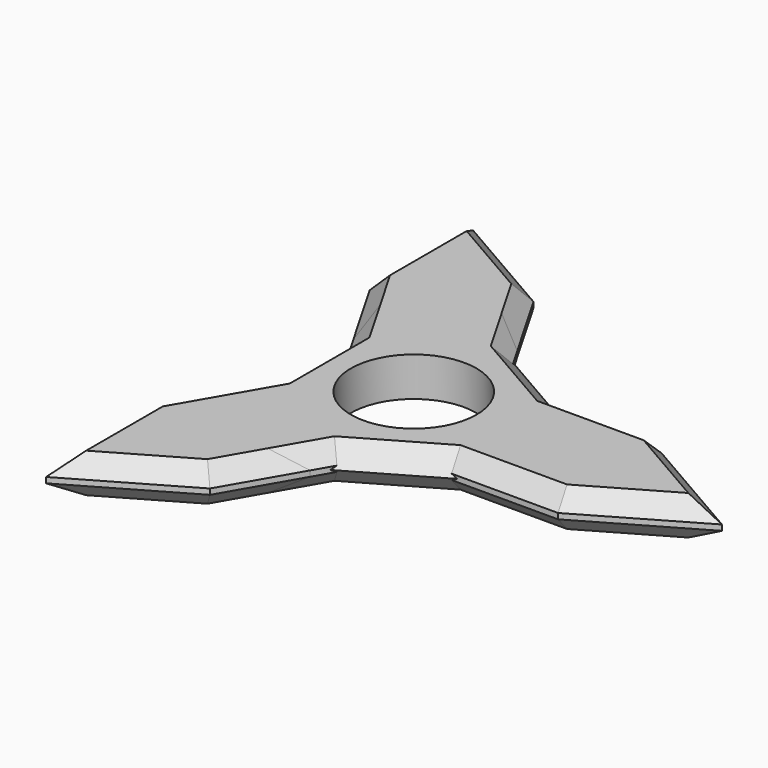
from build123d import *

# Parameters (mm, degrees)
F1_DEPTH      = 7
F2_SIZE       = 3
F3_T4_DEPTH   = 23.0940107676
F3_T10_DEPTH  = 23.0940107676
F3_T16_DEPTH  = 23.0940107676
F3_T22_DEPTH  = 23.0940107676
F3_T28_DEPTH  = 23.0940107676
F3_T34_DEPTH  = 23.0940107676
F3_T40_DEPTH  = 23.0940107676
F3_T46_DEPTH  = 23.0940107676
F3_T52_DEPTH  = 23.0940107676
F3_T58_DEPTH  = 23.0940107676
F3_T64_DEPTH  = 23.0940107676
F3_T70_DEPTH  = 23.0940107676
F3_T76_DEPTH  = 23.0940107676
F3_T82_DEPTH  = 23.0940107676
F3_T88_DEPTH  = 23.0940107676
F3_T94_DEPTH  = 23.0940107676
F3_T100_DEPTH = 23.0940107676
F3_T106_DEPTH = 23.0940107676
F3_T112_DEPTH = 23.0940107676
F3_T118_DEPTH = 23.0940107676
F3_T124_DEPTH = 23.0940107676
F3_T130_DEPTH = 23.0940107676
F3_T136_DEPTH = 23.0940107676
F3_T142_DEPTH = 23.0940107676
F3_T148_DEPTH = 18.8584149398
F3_T153_DEPTH = 18.8584149398
F3_T158_DEPTH = 18.8584149398
F3_T163_DEPTH = 18.8584149398
F3_T168_DEPTH = 18.8584149398
F3_T173_DEPTH = 18.8584149398
F3_T178_DEPTH = 18.8584149398
F3_T183_DEPTH = 18.8584149398
F3_T188_DEPTH = 18.8584149398
F3_T193_DEPTH = 18.8584149398
F3_T198_DEPTH = 18.8584149398
F3_T203_DEPTH = 18.8584149398
F3_T208_DEPTH = 18.8584149398
F3_T213_DEPTH = 18.8584149398
F3_T218_DEPTH = 18.8584149398
F3_T223_DEPTH = 18.8584149398
F3_T228_DEPTH = 18.8584149398
F3_T233_DEPTH = 18.8584149398
F3_T238_DEPTH = 18.8584149398
F3_T243_DEPTH = 18.8584149398
F3_T248_DEPTH = 18.8584149398
F3_T253_DEPTH = 18.8584149398
F3_T258_DEPTH = 18.8584149398
F3_T263_DEPTH = 18.8584149398


# Not quite as in the source:
# - a fillet or chamfer that OpenCascade refuses, or shapes differently, is made with other operations: its cross-section is extruded or revolved along the edge and cut away or added


with BuildPart() as f1:
    # F0 (on Top) → F1 (new body)
    with BuildSketch(Plane.XY):
        Polygon((-20, 11.5470053838), (-20, 0), (-20, -11.5470053838), (0, -23.0940107676), (20, -11.5470053838), (20, 11.5470053838), (0, 23.0940107676), align=None)
        with BuildLine():
            ThreePointArc((-11.2, 0), (0, 11.2), (11.2, 0))
            ThreePointArc((11.2, 0), (0, -11.2), (-11.2, 0))
        make_face(mode=Mode.SUBTRACT)
        Polygon((0, -23.0940107676), (-20, -11.5470053838), (-7.5, -36.0843918244), align=None)
        Polygon((-7.5, -36.0843918244), (-20, -11.5470053838), (-27.5, -24.5373864406), (-17.5, -30.3108891325), align=None)
        Polygon((-27.5, 24.5373864406), (-20, 11.5470053838), (0, 23.0940107676), align=None)
        Polygon((-27.5, -47.6313972081), (-7.5, -36.0843918244), (-17.5, -30.3108891325), align=None)
        Polygon((-17.5, -30.3108891325), (-27.5, -24.5373864406), (-27.5, -47.6313972081), align=None)
        Polygon((-27.5, 24.5373864406), (0, 23.0940107676), (-7.5, 36.0843918244), (-17.5, 30.3108891325), align=None)
        Polygon((-27.5, 47.6313972081), (-27.5, 24.5373864406), (-17.5, 30.3108891325), align=None)
        Polygon((20, 11.5470053838), (20, -11.5470053838), (35, 11.5470053838), align=None)
        Polygon((35, 11.5470053838), (20, -11.5470053838), (35, -11.5470053838), (35, 0), align=None)
        Polygon((-17.5, 30.3108891325), (-7.5, 36.0843918244), (-27.5, 47.6313972081), align=None)
        Polygon((55, 0), (35, 11.5470053838), (35, 0), align=None)
        Polygon((35, 0), (35, -11.5470053838), (55, 0), align=None)
    extrude(amount=F1_DEPTH)

    # F2
    f2_edges = [f1.edges().sort_by_distance(p)[0] for p in [
        (-27.5, 36.084392, 7),
        (-3.75, 29.589201, 7),
        (-23.75, 18.042196, 7),
        (-17.5, 41.857895, 7),
        (27.5, 11.547005, 7),
        (45, 5.773503, 7),
        (45, -5.773503, 7),
        (27.5, -11.547005, 7),
        (-3.75, -29.589201, 7),
        (-17.5, -41.857895, 7),
        (-27.5, -36.084392, 7),
        (-23.75, -18.042196, 7),
        (-17.5, 41.857895, 0),
        (-27.5, 36.084392, 0),
        (-3.75, 29.589201, 0),
        (-23.75, 18.042196, 0),
        (-23.75, -18.042196, 0),
        (-27.5, -36.084392, 0),
        (-17.5, -41.857895, 0),
        (-3.75, -29.589201, 0),
        (27.5, -11.547005, 0),
        (45, -5.773503, 0),
        (45, 5.773503, 0),
        (27.5, 11.547005, 0),
    ]]
    chamfer(f2_edges, length=F2_SIZE)

    # F3: chamfer of 5 on 6 edges, made by hand


with BuildPart() as f3_tool2:
    # F3_s3 → F3_t4 (new body)
    with BuildSketch(Plane(origin=(10, -5.7735026919, 0), x_dir=(0, 0, 1), z_dir=(-0.8660254038, 0.5, 0))):
        Polygon((0, 15), (5, 20), (0, 20), align=None)
    extrude(amount=F3_T4_DEPTH)

    split(bisect_by=Plane(origin=(0, 7.7735026919, 7.7735026919), x_dir=(1, 0, 0), z_dir=(0, 0.7071067812, 0.7071067812)), keep=Keep.TOP)

    split(bisect_by=Plane(origin=(10, 5.7735026919, 0), x_dir=(0, 0, 1), z_dir=(0.8660254038, 0.5, 0)), keep=Keep.TOP)


with BuildPart() as f1_1:
    add(f1.part)

    # F3_t1: cut F3_tool2
    add(f3_tool2.part, mode=Mode.SUBTRACT)


with BuildPart() as f3_tool8:
    # F3_s9 → F3_t10 (new body)
    with BuildSketch(Plane(origin=(10, -5.7735026919, 0), x_dir=(0, 0, 1), z_dir=(-0.8660254038, 0.5, 0))):
        Polygon((0, 15), (5, 20), (0, 20), align=None)
    extrude(amount=F3_T10_DEPTH)

    split(bisect_by=Plane(origin=(3.7009618943, 2.1367513459, -4.2735026919), x_dir=(-0.5, 0.8660254038, 0), z_dir=(0.6123724357, 0.3535533906, -0.7071067812)), keep=Keep.TOP)

    split(bisect_by=Plane.XZ.offset(-11.5470053838), keep=Keep.BOTTOM)


with BuildPart() as f1_2:
    add(f1_1.part)

    # F3_t7: cut F3_tool8
    add(f3_tool8.part, mode=Mode.SUBTRACT)


with BuildPart() as f3_tool14:
    # F3_s15 → F3_t16 (new body)
    with BuildSketch(Plane(origin=(10, -5.7735026919, 0), x_dir=(0, 0, 1), z_dir=(-0.8660254038, 0.5, 0))):
        Polygon((0, 15), (5, 20), (0, 20), align=None)
    extrude(amount=F3_T16_DEPTH)

    split(bisect_by=Plane(origin=(0, 4.2735026919, -4.2735026919), x_dir=(1, 0, 0), z_dir=(0, 0.7071067812, -0.7071067812)), keep=Keep.TOP)

    split(bisect_by=Plane(origin=(10, 5.7735026919, 0), x_dir=(0, 0, 1), z_dir=(0.8660254038, 0.5, 0)), keep=Keep.TOP)


with BuildPart() as f1_3:
    add(f1_2.part)

    # F3_t13: cut F3_tool14
    add(f3_tool14.part, mode=Mode.SUBTRACT)


with BuildPart() as f3_tool20:
    # F3_s21 → F3_t22 (new body)
    with BuildSketch(Plane(origin=(10, -5.7735026919, 0), x_dir=(0, 0, 1), z_dir=(-0.8660254038, 0.5, 0))):
        Polygon((0, 15), (5, 20), (0, 20), align=None)
    extrude(amount=F3_T22_DEPTH)

    split(bisect_by=Plane(origin=(6.7320508076, 3.8867513459, 7.7735026919), x_dir=(-0.5, 0.8660254038, 0), z_dir=(0.6123724357, 0.3535533906, 0.7071067812)), keep=Keep.TOP)

    split(bisect_by=Plane(origin=(10, 5.7735026919, 0), x_dir=(0, 0, 1), z_dir=(-0.8660254038, -0.5, 0)), keep=Keep.TOP)


with BuildPart() as f1_4:
    add(f1_3.part)

    # F3_t19: cut F3_tool20
    add(f3_tool20.part, mode=Mode.SUBTRACT)


with BuildPart() as f3_tool26:
    # F3_s27 → F3_t28 (new body)
    with BuildSketch(Plane.XZ.offset(-11.5470053838)):
        Polygon((-20, 5), (-15, 0), (-20, 0), align=None)
    extrude(amount=F3_T28_DEPTH)

    split(bisect_by=Plane(origin=(-10, -5.7735026919, 0), x_dir=(0, 0, 1), z_dir=(-0.8660254038, -0.5, 0)), keep=Keep.TOP)

    split(bisect_by=Plane(origin=(-10, 5.7735026919, 0), x_dir=(0, 0, 1), z_dir=(-0.8660254038, 0.5, 0)), keep=Keep.TOP)


with BuildPart() as f1_5:
    add(f1_4.part)

    # F3_t25: cut F3_tool26
    add(f3_tool26.part, mode=Mode.SUBTRACT)


with BuildPart() as f3_tool32:
    # F3_s33 → F3_t34 (new body)
    with BuildSketch(Plane.XZ.offset(-11.5470053838)):
        Polygon((-20, 5), (-15, 0), (-20, 0), align=None)
    extrude(amount=F3_T34_DEPTH)

    split(bisect_by=Plane(origin=(-6.7320508076, -3.8867513459, 7.7735026919), x_dir=(0.5, -0.8660254038, 0), z_dir=(-0.6123724357, -0.3535533906, 0.7071067812)), keep=Keep.TOP)

    split(bisect_by=Plane(origin=(-3.7009618943, 2.1367513459, -4.2735026919), x_dir=(-0.5, -0.8660254038, 0), z_dir=(-0.6123724357, 0.3535533906, -0.7071067812)), keep=Keep.TOP)


with BuildPart() as f1_6:
    add(f1_5.part)

    # F3_t31: cut F3_tool32
    add(f3_tool32.part, mode=Mode.SUBTRACT)


with BuildPart() as f3_tool38:
    # F3_s39 → F3_t40 (new body)
    with BuildSketch(Plane.XZ.offset(-11.5470053838)):
        Polygon((-20, 5), (-15, 0), (-20, 0), align=None)
    extrude(amount=F3_T40_DEPTH)

    split(bisect_by=Plane(origin=(-3.7009618943, -2.1367513459, -4.2735026919), x_dir=(0.5, -0.8660254038, 0), z_dir=(-0.6123724357, -0.3535533906, -0.7071067812)), keep=Keep.TOP)

    split(bisect_by=Plane(origin=(-3.7009618943, 2.1367513459, -4.2735026919), x_dir=(-0.5, -0.8660254038, 0), z_dir=(-0.6123724357, 0.3535533906, -0.7071067812)), keep=Keep.TOP)


with BuildPart() as f1_7:
    add(f1_6.part)

    # F3_t37: cut F3_tool38
    add(f3_tool38.part, mode=Mode.SUBTRACT)


with BuildPart() as f3_tool44:
    # F3_s45 → F3_t46 (new body)
    with BuildSketch(Plane.XZ.offset(-11.5470053838)):
        Polygon((-20, 5), (-15, 0), (-20, 0), align=None)
    extrude(amount=F3_T46_DEPTH)

    split(bisect_by=Plane(origin=(-6.7320508076, 3.8867513459, 7.7735026919), x_dir=(-0.5, -0.8660254038, 0), z_dir=(-0.6123724357, 0.3535533906, 0.7071067812)), keep=Keep.TOP)

    split(bisect_by=Plane(origin=(-10, 5.7735026919, 0), x_dir=(0, 0, 1), z_dir=(0.8660254038, -0.5, 0)), keep=Keep.TOP)


with BuildPart() as f1_8:
    add(f1_7.part)

    # F3_t43: cut F3_tool44
    add(f3_tool44.part, mode=Mode.SUBTRACT)


with BuildPart() as f3_tool50:
    # F3_s51 → F3_t52 (new body)
    with BuildSketch(Plane(origin=(-10, -5.7735026919, 0), x_dir=(0, 0, 1), z_dir=(0.8660254038, 0.5, 0))):
        Polygon((0, 15), (5, 20), (0, 20), align=None)
    extrude(amount=F3_T52_DEPTH)

    split(bisect_by=Plane(origin=(6.7320508076, -3.8867513459, 7.7735026919), x_dir=(0.5, 0.8660254038, 0), z_dir=(0.6123724357, -0.3535533906, 0.7071067812)), keep=Keep.TOP)

    split(bisect_by=Plane.XZ.offset(11.5470053838), keep=Keep.TOP)


with BuildPart() as f1_9:
    add(f1_8.part)

    # F3_t49: cut F3_tool50
    add(f3_tool50.part, mode=Mode.SUBTRACT)


with BuildPart() as f3_tool56:
    # F3_s57 → F3_t58 (new body)
    with BuildSketch(Plane(origin=(-10, -5.7735026919, 0), x_dir=(0, 0, 1), z_dir=(0.8660254038, 0.5, 0))):
        Polygon((0, 15), (5, 20), (0, 20), align=None)
    extrude(amount=F3_T58_DEPTH)

    split(bisect_by=Plane(origin=(0, -4.2735026919, -4.2735026919), x_dir=(1, 0, 0), z_dir=(0, -0.7071067812, -0.7071067812)), keep=Keep.TOP)

    split(bisect_by=Plane(origin=(10, -5.7735026919, 0), x_dir=(0, 0, 1), z_dir=(0.8660254038, -0.5, 0)), keep=Keep.TOP)


with BuildPart() as f1_10:
    add(f1_9.part)

    # F3_t55: cut F3_tool56
    add(f3_tool56.part, mode=Mode.SUBTRACT)


with BuildPart() as f3_tool62:
    # F3_s63 → F3_t64 (new body)
    with BuildSketch(Plane(origin=(-10, -5.7735026919, 0), x_dir=(0, 0, 1), z_dir=(0.8660254038, 0.5, 0))):
        Polygon((0, 15), (5, 20), (0, 20), align=None)
    extrude(amount=F3_T64_DEPTH)

    split(bisect_by=Plane(origin=(3.7009618943, -2.1367513459, -4.2735026919), x_dir=(0.5, 0.8660254038, 0), z_dir=(0.6123724357, -0.3535533906, -0.7071067812)), keep=Keep.TOP)

    split(bisect_by=Plane(origin=(10, -5.7735026919, 0), x_dir=(0, 0, 1), z_dir=(-0.8660254038, 0.5, 0)), keep=Keep.TOP)


with BuildPart() as f1_11:
    add(f1_10.part)

    # F3_t61: cut F3_tool62
    add(f3_tool62.part, mode=Mode.SUBTRACT)


with BuildPart() as f3_tool68:
    # F3_s69 → F3_t70 (new body)
    with BuildSketch(Plane(origin=(-10, -5.7735026919, 0), x_dir=(0, 0, 1), z_dir=(0.8660254038, 0.5, 0))):
        Polygon((0, 15), (5, 20), (0, 20), align=None)
    extrude(amount=F3_T70_DEPTH)

    split(bisect_by=Plane(origin=(0, -7.7735026919, 7.7735026919), x_dir=(1, 0, 0), z_dir=(0, -0.7071067812, 0.7071067812)), keep=Keep.TOP)

    split(bisect_by=Plane(origin=(10, -5.7735026919, 0), x_dir=(0, 0, 1), z_dir=(0.8660254038, -0.5, 0)), keep=Keep.TOP)


with BuildPart() as f1_12:
    add(f1_11.part)

    # F3_t67: cut F3_tool68
    add(f3_tool68.part, mode=Mode.SUBTRACT)


with BuildPart() as f3_tool74:
    # F3_s75 → F3_t76 (new body)
    with BuildSketch(Plane.XZ.offset(-11.5470053838)):
        Polygon((-20, 2), (-15, 7), (-20, 7), align=None)
    extrude(amount=F3_T76_DEPTH)

    split(bisect_by=Plane(origin=(-10, -5.7735026919, 0), x_dir=(0, 0, 1), z_dir=(-0.8660254038, -0.5, 0)), keep=Keep.TOP)

    split(bisect_by=Plane(origin=(-10, 5.7735026919, 0), x_dir=(0, 0, 1), z_dir=(-0.8660254038, 0.5, 0)), keep=Keep.TOP)


with BuildPart() as f1_13:
    add(f1_12.part)

    # F3_t73: cut F3_tool74
    add(f3_tool74.part, mode=Mode.SUBTRACT)


with BuildPart() as f3_tool80:
    # F3_s81 → F3_t82 (new body)
    with BuildSketch(Plane.XZ.offset(-11.5470053838)):
        Polygon((-20, 2), (-15, 7), (-20, 7), align=None)
    extrude(amount=F3_T82_DEPTH)

    split(bisect_by=Plane(origin=(-3.7009618943, -2.1367513459, -4.2735026919), x_dir=(0.5, -0.8660254038, 0), z_dir=(-0.6123724357, -0.3535533906, -0.7071067812)), keep=Keep.TOP)

    split(bisect_by=Plane(origin=(-6.7320508076, 3.8867513459, 7.7735026919), x_dir=(-0.5, -0.8660254038, 0), z_dir=(-0.6123724357, 0.3535533906, 0.7071067812)), keep=Keep.TOP)


with BuildPart() as f1_14:
    add(f1_13.part)

    # F3_t79: cut F3_tool80
    add(f3_tool80.part, mode=Mode.SUBTRACT)


with BuildPart() as f3_tool86:
    # F3_s87 → F3_t88 (new body)
    with BuildSketch(Plane.XZ.offset(-11.5470053838)):
        Polygon((-20, 2), (-15, 7), (-20, 7), align=None)
    extrude(amount=F3_T88_DEPTH)

    split(bisect_by=Plane(origin=(-6.7320508076, -3.8867513459, 7.7735026919), x_dir=(0.5, -0.8660254038, 0), z_dir=(-0.6123724357, -0.3535533906, 0.7071067812)), keep=Keep.TOP)

    split(bisect_by=Plane(origin=(-6.7320508076, 3.8867513459, 7.7735026919), x_dir=(-0.5, -0.8660254038, 0), z_dir=(-0.6123724357, 0.3535533906, 0.7071067812)), keep=Keep.TOP)


with BuildPart() as f1_15:
    add(f1_14.part)

    # F3_t85: cut F3_tool86
    add(f3_tool86.part, mode=Mode.SUBTRACT)


with BuildPart() as f3_tool92:
    # F3_s93 → F3_t94 (new body)
    with BuildSketch(Plane.XZ.offset(-11.5470053838)):
        Polygon((-20, 2), (-15, 7), (-20, 7), align=None)
    extrude(amount=F3_T94_DEPTH)

    split(bisect_by=Plane(origin=(-3.7009618943, 2.1367513459, -4.2735026919), x_dir=(-0.5, -0.8660254038, 0), z_dir=(-0.6123724357, 0.3535533906, -0.7071067812)), keep=Keep.TOP)

    split(bisect_by=Plane(origin=(-10, 5.7735026919, 0), x_dir=(0, 0, 1), z_dir=(0.8660254038, -0.5, 0)), keep=Keep.TOP)


with BuildPart() as f1_16:
    add(f1_15.part)

    # F3_t91: cut F3_tool92
    add(f3_tool92.part, mode=Mode.SUBTRACT)


with BuildPart() as f3_tool98:
    # F3_s99 → F3_t100 (new body)
    with BuildSketch(Plane(origin=(10, -5.7735026919, 0), x_dir=(0, 0, 1), z_dir=(-0.8660254038, 0.5, 0))):
        Polygon((7, 15), (2, 20), (7, 20), align=None)
    extrude(amount=F3_T100_DEPTH)

    split(bisect_by=Plane(origin=(0, 4.2735026919, -4.2735026919), x_dir=(1, 0, 0), z_dir=(0, 0.7071067812, -0.7071067812)), keep=Keep.TOP)

    split(bisect_by=Plane(origin=(10, 5.7735026919, 0), x_dir=(0, 0, 1), z_dir=(0.8660254038, 0.5, 0)), keep=Keep.TOP)


with BuildPart() as f1_17:
    add(f1_16.part)

    # F3_t97: cut F3_tool98
    add(f3_tool98.part, mode=Mode.SUBTRACT)


with BuildPart() as f3_tool104:
    # F3_s105 → F3_t106 (new body)
    with BuildSketch(Plane(origin=(10, -5.7735026919, 0), x_dir=(0, 0, 1), z_dir=(-0.8660254038, 0.5, 0))):
        Polygon((7, 15), (2, 20), (7, 20), align=None)
    extrude(amount=F3_T106_DEPTH)

    split(bisect_by=Plane(origin=(6.7320508076, 3.8867513459, 7.7735026919), x_dir=(-0.5, 0.8660254038, 0), z_dir=(0.6123724357, 0.3535533906, 0.7071067812)), keep=Keep.TOP)

    split(bisect_by=Plane.XZ.offset(-11.5470053838), keep=Keep.BOTTOM)


with BuildPart() as f1_18:
    add(f1_17.part)

    # F3_t103: cut F3_tool104
    add(f3_tool104.part, mode=Mode.SUBTRACT)


with BuildPart() as f3_tool110:
    # F3_s111 → F3_t112 (new body)
    with BuildSketch(Plane(origin=(10, -5.7735026919, 0), x_dir=(0, 0, 1), z_dir=(-0.8660254038, 0.5, 0))):
        Polygon((7, 15), (2, 20), (7, 20), align=None)
    extrude(amount=F3_T112_DEPTH)

    split(bisect_by=Plane(origin=(0, 7.7735026919, 7.7735026919), x_dir=(1, 0, 0), z_dir=(0, 0.7071067812, 0.7071067812)), keep=Keep.TOP)

    split(bisect_by=Plane(origin=(10, 5.7735026919, 0), x_dir=(0, 0, 1), z_dir=(0.8660254038, 0.5, 0)), keep=Keep.TOP)


with BuildPart() as f1_19:
    add(f1_18.part)

    # F3_t109: cut F3_tool110
    add(f3_tool110.part, mode=Mode.SUBTRACT)


with BuildPart() as f3_tool116:
    # F3_s117 → F3_t118 (new body)
    with BuildSketch(Plane(origin=(10, -5.7735026919, 0), x_dir=(0, 0, 1), z_dir=(-0.8660254038, 0.5, 0))):
        Polygon((7, 15), (2, 20), (7, 20), align=None)
    extrude(amount=F3_T118_DEPTH)

    split(bisect_by=Plane(origin=(3.7009618943, 2.1367513459, -4.2735026919), x_dir=(-0.5, 0.8660254038, 0), z_dir=(0.6123724357, 0.3535533906, -0.7071067812)), keep=Keep.TOP)

    split(bisect_by=Plane(origin=(10, 5.7735026919, 0), x_dir=(0, 0, 1), z_dir=(-0.8660254038, -0.5, 0)), keep=Keep.TOP)


with BuildPart() as f1_20:
    add(f1_19.part)

    # F3_t115: cut F3_tool116
    add(f3_tool116.part, mode=Mode.SUBTRACT)


with BuildPart() as f3_tool122:
    # F3_s123 → F3_t124 (new body)
    with BuildSketch(Plane(origin=(-10, -5.7735026919, 0), x_dir=(0, 0, 1), z_dir=(0.8660254038, 0.5, 0))):
        Polygon((7, 15), (2, 20), (7, 20), align=None)
    extrude(amount=F3_T124_DEPTH)

    split(bisect_by=Plane(origin=(3.7009618943, -2.1367513459, -4.2735026919), x_dir=(0.5, 0.8660254038, 0), z_dir=(0.6123724357, -0.3535533906, -0.7071067812)), keep=Keep.TOP)

    split(bisect_by=Plane.XZ.offset(11.5470053838), keep=Keep.TOP)


with BuildPart() as f1_21:
    add(f1_20.part)

    # F3_t121: cut F3_tool122
    add(f3_tool122.part, mode=Mode.SUBTRACT)


with BuildPart() as f3_tool128:
    # F3_s129 → F3_t130 (new body)
    with BuildSketch(Plane(origin=(-10, -5.7735026919, 0), x_dir=(0, 0, 1), z_dir=(0.8660254038, 0.5, 0))):
        Polygon((7, 15), (2, 20), (7, 20), align=None)
    extrude(amount=F3_T130_DEPTH)

    split(bisect_by=Plane(origin=(0, -7.7735026919, 7.7735026919), x_dir=(1, 0, 0), z_dir=(0, -0.7071067812, 0.7071067812)), keep=Keep.TOP)

    split(bisect_by=Plane(origin=(10, -5.7735026919, 0), x_dir=(0, 0, 1), z_dir=(0.8660254038, -0.5, 0)), keep=Keep.TOP)


with BuildPart() as f1_22:
    add(f1_21.part)

    # F3_t127: cut F3_tool128
    add(f3_tool128.part, mode=Mode.SUBTRACT)


with BuildPart() as f3_tool134:
    # F3_s135 → F3_t136 (new body)
    with BuildSketch(Plane(origin=(-10, -5.7735026919, 0), x_dir=(0, 0, 1), z_dir=(0.8660254038, 0.5, 0))):
        Polygon((7, 15), (2, 20), (7, 20), align=None)
    extrude(amount=F3_T136_DEPTH)

    split(bisect_by=Plane(origin=(6.7320508076, -3.8867513459, 7.7735026919), x_dir=(0.5, 0.8660254038, 0), z_dir=(0.6123724357, -0.3535533906, 0.7071067812)), keep=Keep.TOP)

    split(bisect_by=Plane(origin=(10, -5.7735026919, 0), x_dir=(0, 0, 1), z_dir=(-0.8660254038, 0.5, 0)), keep=Keep.TOP)


with BuildPart() as f1_23:
    add(f1_22.part)

    # F3_t133: cut F3_tool134
    add(f3_tool134.part, mode=Mode.SUBTRACT)


with BuildPart() as f3_tool140:
    # F3_s141 → F3_t142 (new body)
    with BuildSketch(Plane(origin=(-10, -5.7735026919, 0), x_dir=(0, 0, 1), z_dir=(0.8660254038, 0.5, 0))):
        Polygon((7, 15), (2, 20), (7, 20), align=None)
    extrude(amount=F3_T142_DEPTH)

    split(bisect_by=Plane(origin=(0, -4.2735026919, -4.2735026919), x_dir=(1, 0, 0), z_dir=(0, -0.7071067812, -0.7071067812)), keep=Keep.TOP)

    split(bisect_by=Plane(origin=(10, -5.7735026919, 0), x_dir=(0, 0, 1), z_dir=(0.8660254038, -0.5, 0)), keep=Keep.TOP)


with BuildPart() as f1_24:
    add(f1_23.part)

    # F3_t139: cut F3_tool140
    add(f3_tool140.part, mode=Mode.SUBTRACT)


with BuildPart() as f3_tool146:
    # F3_s147 → F3_t148 (new body)
    with BuildSketch(Plane(origin=(-10, -5.7735026919, 0), x_dir=(0, 0, 1), z_dir=(-0.8660254038, -0.5, 0))):
        Polygon((7, -15), (2, -20), (7, -20), align=None)
    extrude(amount=F3_T148_DEPTH)

    split(bisect_by=Plane(origin=(3.7009618943, -2.1367513459, -4.2735026919), x_dir=(0.5, 0.8660254038, 0), z_dir=(0.6123724357, -0.3535533906, -0.7071067812)), keep=Keep.TOP)


with BuildPart() as f1_25:
    add(f1_24.part)

    # F3_t145: cut F3_tool146
    add(f3_tool146.part, mode=Mode.SUBTRACT)


with BuildPart() as f3_tool151:
    # F3_s152 → F3_t153 (new body)
    with BuildSketch(Plane(origin=(-10, -5.7735026919, 0), x_dir=(0, 0, 1), z_dir=(-0.8660254038, -0.5, 0))):
        Polygon((7, -15), (2, -20), (7, -20), align=None)
    extrude(amount=F3_T153_DEPTH)

    split(bisect_by=Plane(origin=(6.7320508076, -3.8867513459, 7.7735026919), x_dir=(0.5, 0.8660254038, 0), z_dir=(0.6123724357, -0.3535533906, 0.7071067812)), keep=Keep.TOP)


with BuildPart() as f1_26:
    add(f1_25.part)

    # F3_t150: cut F3_tool151
    add(f3_tool151.part, mode=Mode.SUBTRACT)


with BuildPart() as f3_tool156:
    # F3_s157 → F3_t158 (new body)
    with BuildSketch(Plane(origin=(10, 5.7735026919, 0), x_dir=(0, 0, 1), z_dir=(0.8660254038, 0.5, 0))):
        Polygon((7, 15), (2, 20), (7, 20), align=None)
    extrude(amount=F3_T158_DEPTH)

    split(bisect_by=Plane(origin=(0, -4.2735026919, -4.2735026919), x_dir=(1, 0, 0), z_dir=(0, -0.7071067812, -0.7071067812)), keep=Keep.TOP)


with BuildPart() as f1_27:
    add(f1_26.part)

    # F3_t155: cut F3_tool156
    add(f3_tool156.part, mode=Mode.SUBTRACT)


with BuildPart() as f3_tool161:
    # F3_s162 → F3_t163 (new body)
    with BuildSketch(Plane(origin=(10, 5.7735026919, 0), x_dir=(0, 0, 1), z_dir=(0.8660254038, 0.5, 0))):
        Polygon((7, 15), (2, 20), (7, 20), align=None)
    extrude(amount=F3_T163_DEPTH)

    split(bisect_by=Plane(origin=(0, -7.7735026919, 7.7735026919), x_dir=(1, 0, 0), z_dir=(0, -0.7071067812, 0.7071067812)), keep=Keep.TOP)


with BuildPart() as f1_28:
    add(f1_27.part)

    # F3_t160: cut F3_tool161
    add(f3_tool161.part, mode=Mode.SUBTRACT)


with BuildPart() as f3_tool166:
    # F3_s167 → F3_t168 (new body)
    with BuildSketch(Plane(origin=(10, -5.7735026919, 0), x_dir=(0, 0, 1), z_dir=(0.8660254038, -0.5, 0))):
        Polygon((7, -15), (2, -20), (7, -20), align=None)
    extrude(amount=F3_T168_DEPTH)

    split(bisect_by=Plane(origin=(0, 4.2735026919, -4.2735026919), x_dir=(1, 0, 0), z_dir=(0, 0.7071067812, -0.7071067812)), keep=Keep.TOP)


with BuildPart() as f1_29:
    add(f1_28.part)

    # F3_t165: cut F3_tool166
    add(f3_tool166.part, mode=Mode.SUBTRACT)


with BuildPart() as f3_tool171:
    # F3_s172 → F3_t173 (new body)
    with BuildSketch(Plane(origin=(10, -5.7735026919, 0), x_dir=(0, 0, 1), z_dir=(0.8660254038, -0.5, 0))):
        Polygon((7, -15), (2, -20), (7, -20), align=None)
    extrude(amount=F3_T173_DEPTH)

    split(bisect_by=Plane(origin=(0, 7.7735026919, 7.7735026919), x_dir=(1, 0, 0), z_dir=(0, 0.7071067812, 0.7071067812)), keep=Keep.TOP)


with BuildPart() as f1_30:
    add(f1_29.part)

    # F3_t170: cut F3_tool171
    add(f3_tool171.part, mode=Mode.SUBTRACT)


with BuildPart() as f3_tool176:
    # F3_s177 → F3_t178 (new body)
    with BuildSketch(Plane(origin=(-10, 5.7735026919, 0), x_dir=(0, 0, 1), z_dir=(-0.8660254038, 0.5, 0))):
        Polygon((7, 15), (2, 20), (7, 20), align=None)
    extrude(amount=F3_T178_DEPTH)

    split(bisect_by=Plane(origin=(3.7009618943, 2.1367513459, -4.2735026919), x_dir=(-0.5, 0.8660254038, 0), z_dir=(0.6123724357, 0.3535533906, -0.7071067812)), keep=Keep.TOP)


with BuildPart() as f1_31:
    add(f1_30.part)

    # F3_t175: cut F3_tool176
    add(f3_tool176.part, mode=Mode.SUBTRACT)


with BuildPart() as f3_tool181:
    # F3_s182 → F3_t183 (new body)
    with BuildSketch(Plane(origin=(-10, 5.7735026919, 0), x_dir=(0, 0, 1), z_dir=(-0.8660254038, 0.5, 0))):
        Polygon((7, 15), (2, 20), (7, 20), align=None)
    extrude(amount=F3_T183_DEPTH)

    split(bisect_by=Plane(origin=(6.7320508076, 3.8867513459, 7.7735026919), x_dir=(-0.5, 0.8660254038, 0), z_dir=(0.6123724357, 0.3535533906, 0.7071067812)), keep=Keep.TOP)


with BuildPart() as f1_32:
    add(f1_31.part)

    # F3_t180: cut F3_tool181
    add(f3_tool181.part, mode=Mode.SUBTRACT)


with BuildPart() as f3_tool186:
    # F3_s187 → F3_t188 (new body)
    with BuildSketch(Plane.XZ.offset(-11.5470053838)):
        Polygon((-20, 2), (-15, 7), (-20, 7), align=None)
    extrude(amount=-F3_T188_DEPTH)

    split(bisect_by=Plane(origin=(-3.7009618943, -2.1367513459, -4.2735026919), x_dir=(0.5, -0.8660254038, 0), z_dir=(-0.6123724357, -0.3535533906, -0.7071067812)), keep=Keep.TOP)


with BuildPart() as f1_33:
    add(f1_32.part)

    # F3_t185: cut F3_tool186
    add(f3_tool186.part, mode=Mode.SUBTRACT)


with BuildPart() as f3_tool191:
    # F3_s192 → F3_t193 (new body)
    with BuildSketch(Plane.XZ.offset(-11.5470053838)):
        Polygon((-20, 2), (-15, 7), (-20, 7), align=None)
    extrude(amount=-F3_T193_DEPTH)

    split(bisect_by=Plane(origin=(-6.7320508076, -3.8867513459, 7.7735026919), x_dir=(0.5, -0.8660254038, 0), z_dir=(-0.6123724357, -0.3535533906, 0.7071067812)), keep=Keep.TOP)


with BuildPart() as f1_34:
    add(f1_33.part)

    # F3_t190: cut F3_tool191
    add(f3_tool191.part, mode=Mode.SUBTRACT)


with BuildPart() as f3_tool196:
    # F3_s197 → F3_t198 (new body)
    with BuildSketch(Plane.XZ.offset(11.5470053838)):
        Polygon((-20, 2), (-15, 7), (-20, 7), align=None)
    extrude(amount=F3_T198_DEPTH)

    split(bisect_by=Plane(origin=(-3.7009618943, 2.1367513459, -4.2735026919), x_dir=(-0.5, -0.8660254038, 0), z_dir=(-0.6123724357, 0.3535533906, -0.7071067812)), keep=Keep.TOP)


with BuildPart() as f1_35:
    add(f1_34.part)

    # F3_t195: cut F3_tool196
    add(f3_tool196.part, mode=Mode.SUBTRACT)


with BuildPart() as f3_tool201:
    # F3_s202 → F3_t203 (new body)
    with BuildSketch(Plane.XZ.offset(11.5470053838)):
        Polygon((-20, 2), (-15, 7), (-20, 7), align=None)
    extrude(amount=F3_T203_DEPTH)

    split(bisect_by=Plane(origin=(-6.7320508076, 3.8867513459, 7.7735026919), x_dir=(-0.5, -0.8660254038, 0), z_dir=(-0.6123724357, 0.3535533906, 0.7071067812)), keep=Keep.TOP)


with BuildPart() as f1_36:
    add(f1_35.part)

    # F3_t200: cut F3_tool201
    add(f3_tool201.part, mode=Mode.SUBTRACT)


with BuildPart() as f3_tool206:
    # F3_s207 → F3_t208 (new body)
    with BuildSketch(Plane(origin=(-10, -5.7735026919, 0), x_dir=(0, 0, 1), z_dir=(-0.8660254038, -0.5, 0))):
        Polygon((0, -15), (5, -20), (0, -20), align=None)
    extrude(amount=F3_T208_DEPTH)

    split(bisect_by=Plane(origin=(6.7320508076, -3.8867513459, 7.7735026919), x_dir=(0.5, 0.8660254038, 0), z_dir=(0.6123724357, -0.3535533906, 0.7071067812)), keep=Keep.TOP)


with BuildPart() as f1_37:
    add(f1_36.part)

    # F3_t205: cut F3_tool206
    add(f3_tool206.part, mode=Mode.SUBTRACT)


with BuildPart() as f3_tool211:
    # F3_s212 → F3_t213 (new body)
    with BuildSketch(Plane(origin=(-10, -5.7735026919, 0), x_dir=(0, 0, 1), z_dir=(-0.8660254038, -0.5, 0))):
        Polygon((0, -15), (5, -20), (0, -20), align=None)
    extrude(amount=F3_T213_DEPTH)

    split(bisect_by=Plane(origin=(3.7009618943, -2.1367513459, -4.2735026919), x_dir=(0.5, 0.8660254038, 0), z_dir=(0.6123724357, -0.3535533906, -0.7071067812)), keep=Keep.TOP)


with BuildPart() as f1_38:
    add(f1_37.part)

    # F3_t210: cut F3_tool211
    add(f3_tool211.part, mode=Mode.SUBTRACT)


with BuildPart() as f3_tool216:
    # F3_s217 → F3_t218 (new body)
    with BuildSketch(Plane(origin=(10, 5.7735026919, 0), x_dir=(0, 0, 1), z_dir=(0.8660254038, 0.5, 0))):
        Polygon((0, 15), (5, 20), (0, 20), align=None)
    extrude(amount=F3_T218_DEPTH)

    split(bisect_by=Plane(origin=(0, -7.7735026919, 7.7735026919), x_dir=(1, 0, 0), z_dir=(0, -0.7071067812, 0.7071067812)), keep=Keep.TOP)


with BuildPart() as f1_39:
    add(f1_38.part)

    # F3_t215: cut F3_tool216
    add(f3_tool216.part, mode=Mode.SUBTRACT)


with BuildPart() as f3_tool221:
    # F3_s222 → F3_t223 (new body)
    with BuildSketch(Plane(origin=(10, 5.7735026919, 0), x_dir=(0, 0, 1), z_dir=(0.8660254038, 0.5, 0))):
        Polygon((0, 15), (5, 20), (0, 20), align=None)
    extrude(amount=F3_T223_DEPTH)

    split(bisect_by=Plane(origin=(0, -4.2735026919, -4.2735026919), x_dir=(1, 0, 0), z_dir=(0, -0.7071067812, -0.7071067812)), keep=Keep.TOP)


with BuildPart() as f1_40:
    add(f1_39.part)

    # F3_t220: cut F3_tool221
    add(f3_tool221.part, mode=Mode.SUBTRACT)


with BuildPart() as f3_tool226:
    # F3_s227 → F3_t228 (new body)
    with BuildSketch(Plane.XZ.offset(-11.5470053838)):
        Polygon((-20, 5), (-15, 0), (-20, 0), align=None)
    extrude(amount=-F3_T228_DEPTH)

    split(bisect_by=Plane(origin=(-6.7320508076, -3.8867513459, 7.7735026919), x_dir=(0.5, -0.8660254038, 0), z_dir=(-0.6123724357, -0.3535533906, 0.7071067812)), keep=Keep.TOP)


with BuildPart() as f1_41:
    add(f1_40.part)

    # F3_t225: cut F3_tool226
    add(f3_tool226.part, mode=Mode.SUBTRACT)


with BuildPart() as f3_tool231:
    # F3_s232 → F3_t233 (new body)
    with BuildSketch(Plane.XZ.offset(-11.5470053838)):
        Polygon((-20, 5), (-15, 0), (-20, 0), align=None)
    extrude(amount=-F3_T233_DEPTH)

    split(bisect_by=Plane(origin=(-3.7009618943, -2.1367513459, -4.2735026919), x_dir=(0.5, -0.8660254038, 0), z_dir=(-0.6123724357, -0.3535533906, -0.7071067812)), keep=Keep.TOP)


with BuildPart() as f1_42:
    add(f1_41.part)

    # F3_t230: cut F3_tool231
    add(f3_tool231.part, mode=Mode.SUBTRACT)


with BuildPart() as f3_tool236:
    # F3_s237 → F3_t238 (new body)
    with BuildSketch(Plane.XZ.offset(11.5470053838)):
        Polygon((-20, 5), (-15, 0), (-20, 0), align=None)
    extrude(amount=F3_T238_DEPTH)

    split(bisect_by=Plane(origin=(-6.7320508076, 3.8867513459, 7.7735026919), x_dir=(-0.5, -0.8660254038, 0), z_dir=(-0.6123724357, 0.3535533906, 0.7071067812)), keep=Keep.TOP)


with BuildPart() as f1_43:
    add(f1_42.part)

    # F3_t235: cut F3_tool236
    add(f3_tool236.part, mode=Mode.SUBTRACT)


with BuildPart() as f3_tool241:
    # F3_s242 → F3_t243 (new body)
    with BuildSketch(Plane.XZ.offset(11.5470053838)):
        Polygon((-20, 5), (-15, 0), (-20, 0), align=None)
    extrude(amount=F3_T243_DEPTH)

    split(bisect_by=Plane(origin=(-3.7009618943, 2.1367513459, -4.2735026919), x_dir=(-0.5, -0.8660254038, 0), z_dir=(-0.6123724357, 0.3535533906, -0.7071067812)), keep=Keep.TOP)


with BuildPart() as f1_44:
    add(f1_43.part)

    # F3_t240: cut F3_tool241
    add(f3_tool241.part, mode=Mode.SUBTRACT)


with BuildPart() as f3_tool246:
    # F3_s247 → F3_t248 (new body)
    with BuildSketch(Plane(origin=(10, -5.7735026919, 0), x_dir=(0, 0, 1), z_dir=(0.8660254038, -0.5, 0))):
        Polygon((0, -15), (5, -20), (0, -20), align=None)
    extrude(amount=F3_T248_DEPTH)

    split(bisect_by=Plane(origin=(0, 7.7735026919, 7.7735026919), x_dir=(1, 0, 0), z_dir=(0, 0.7071067812, 0.7071067812)), keep=Keep.TOP)


with BuildPart() as f1_45:
    add(f1_44.part)

    # F3_t245: cut F3_tool246
    add(f3_tool246.part, mode=Mode.SUBTRACT)


with BuildPart() as f3_tool251:
    # F3_s252 → F3_t253 (new body)
    with BuildSketch(Plane(origin=(10, -5.7735026919, 0), x_dir=(0, 0, 1), z_dir=(0.8660254038, -0.5, 0))):
        Polygon((0, -15), (5, -20), (0, -20), align=None)
    extrude(amount=F3_T253_DEPTH)

    split(bisect_by=Plane(origin=(0, 4.2735026919, -4.2735026919), x_dir=(1, 0, 0), z_dir=(0, 0.7071067812, -0.7071067812)), keep=Keep.TOP)


with BuildPart() as f1_46:
    add(f1_45.part)

    # F3_t250: cut F3_tool251
    add(f3_tool251.part, mode=Mode.SUBTRACT)


with BuildPart() as f3_tool256:
    # F3_s257 → F3_t258 (new body)
    with BuildSketch(Plane(origin=(-10, 5.7735026919, 0), x_dir=(0, 0, 1), z_dir=(-0.8660254038, 0.5, 0))):
        Polygon((0, 15), (5, 20), (0, 20), align=None)
    extrude(amount=F3_T258_DEPTH)

    split(bisect_by=Plane(origin=(6.7320508076, 3.8867513459, 7.7735026919), x_dir=(-0.5, 0.8660254038, 0), z_dir=(0.6123724357, 0.3535533906, 0.7071067812)), keep=Keep.TOP)


with BuildPart() as f1_47:
    add(f1_46.part)

    # F3_t255: cut F3_tool256
    add(f3_tool256.part, mode=Mode.SUBTRACT)


with BuildPart() as f3_tool261:
    # F3_s262 → F3_t263 (new body)
    with BuildSketch(Plane(origin=(-10, 5.7735026919, 0), x_dir=(0, 0, 1), z_dir=(-0.8660254038, 0.5, 0))):
        Polygon((0, 15), (5, 20), (0, 20), align=None)
    extrude(amount=F3_T263_DEPTH)

    split(bisect_by=Plane(origin=(3.7009618943, 2.1367513459, -4.2735026919), x_dir=(-0.5, 0.8660254038, 0), z_dir=(0.6123724357, 0.3535533906, -0.7071067812)), keep=Keep.TOP)


with BuildPart() as f1_48:
    add(f1_47.part)

    # F3_t260: cut F3_tool261
    add(f3_tool261.part, mode=Mode.SUBTRACT)


solid = f1_48.part
